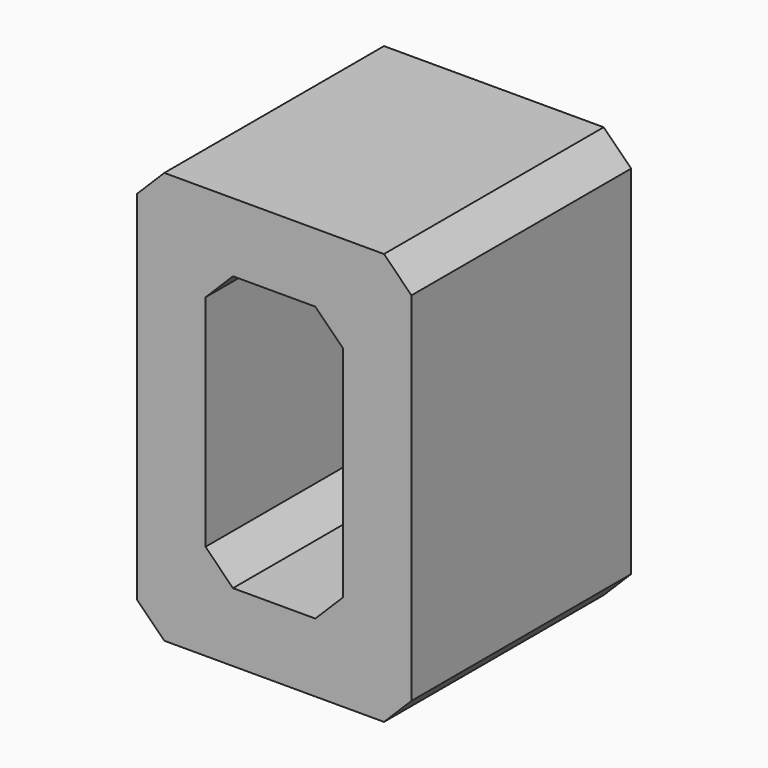
from build123d import *

# Parameters (mm, degrees)
F0_W     = 20
F0_H     = 30
F0_W_2   = 10
F0_H_2   = 20
F1_DEPTH = 20
F2_SIZE  = 2


with BuildPart() as f1:
    # F0 (on Front) → F1 (new body)
    with BuildSketch(Plane.XZ):
        with Locations((10, 15)):
            Rectangle(F0_W, F0_H)
        with Locations((10, 15)):
            Rectangle(F0_W_2, F0_H_2, mode=Mode.SUBTRACT)
    extrude(amount=F1_DEPTH)

    # F2
    f2_edges = [f1.edges().sort_by_distance(p)[0] for p in [
        (0, -10, 30),
        (0, -10, 0),
        (5, -10, 25),
        (5, -10, 5),
        (20, -10, 0),
        (20, -10, 30),
        (15, -10, 25),
        (15, -10, 5),
    ]]
    chamfer(f2_edges, length=F2_SIZE)


solid = f1.part
